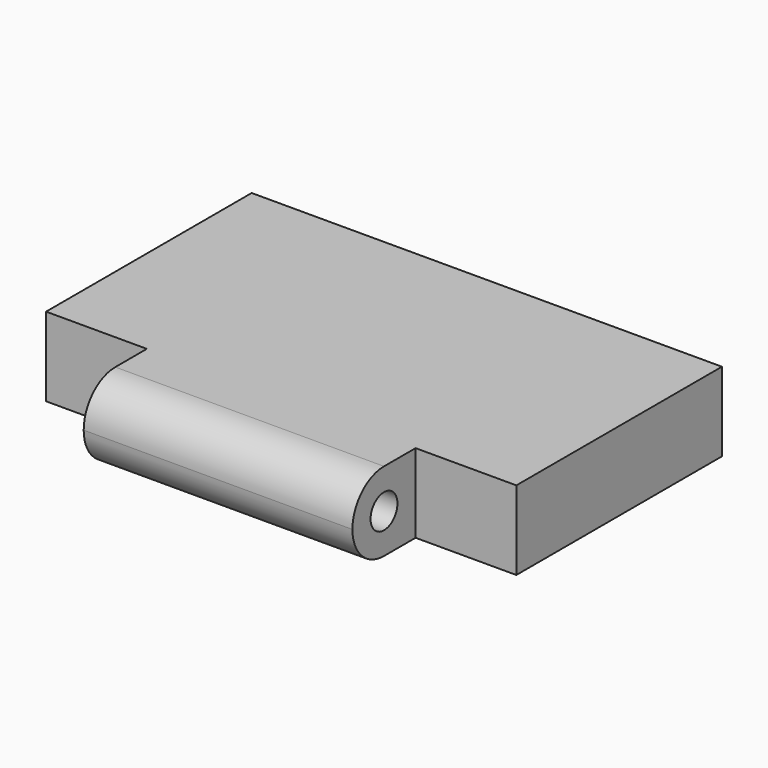
from build123d import *

# Parameters (mm, degrees)
F0_W     = 140
F0_H     = 23.5
F1_DEPTH = 50
F2_R     = 11.74999
F3_R     = 5
F4_DEPTH = 140
F6_DEPTH = 25
F7_W     = 140
F7_H     = 23.5
F8_DEPTH = 50


# Not quite as in the source:
# - a fillet or chamfer is up to 0.001 mm smaller than in the source, because OpenCascade refuses the exact size


with BuildPart() as f1:
    # F0 (on Front) → F1 (new body)
    with BuildSketch(Plane.XZ):
        with Locations((-8.7296748534, -19.8372076215)):
            Rectangle(F0_W, F0_H)
    extrude(amount=F1_DEPTH)

    # F2 (radius 11.75 in the source; OpenCascade refuses exactly that, so slightly less here)
    f2_edges = [f1.edges().sort_by_distance(p)[0] for p in [
        (-8.729675, -50, -8.087208),
        (-8.729675, -50, -31.587208),
    ]]
    fillet(f2_edges, radius=F2_R)

    # F3 (on face) → F4 (cut, through all)
    with BuildSketch(Plane(origin=(-78.7296748534, 0, 0), x_dir=(0, -1, 0), z_dir=(-1, 0, 0))):
        with Locations((38.25, -19.8372076215)):
            Circle(F3_R)
    extrude(amount=-F4_DEPTH, mode=Mode.SUBTRACT)

    # F5 (on face) → F6 (cut)
    with BuildSketch(Plane(origin=(0, 0, -31.5872076215), x_dir=(1, 0, 0), z_dir=(0, 0, -1))):
        Polygon((-48.7296748534, 26.5), (-48.7296748534, 51.5), (-48.7296748534, 66.3150921464), (-82.7311202884, 66.3150921464), (-82.7311202884, 26.5), (-78.7296748534, 26.5), align=None)
        Polygon((31.2703251466, 61.9400218129), (31.2703251466, 51.5), (31.2703251466, 26.5), (74.6265202761, 26.5), (74.6265202761, 61.9400218129), align=None)
    extrude(amount=-F6_DEPTH, mode=Mode.SUBTRACT)

    # F7 (on face) → F8 (join)
    with BuildSketch(Plane(origin=(0, 0, 0), x_dir=(-1, 0, 0), z_dir=(0, 1, 0))):
        with Locations((8.7296748534, -19.8372076215)):
            Rectangle(F7_W, F7_H)
    extrude(amount=F8_DEPTH)


solid = f1.part
